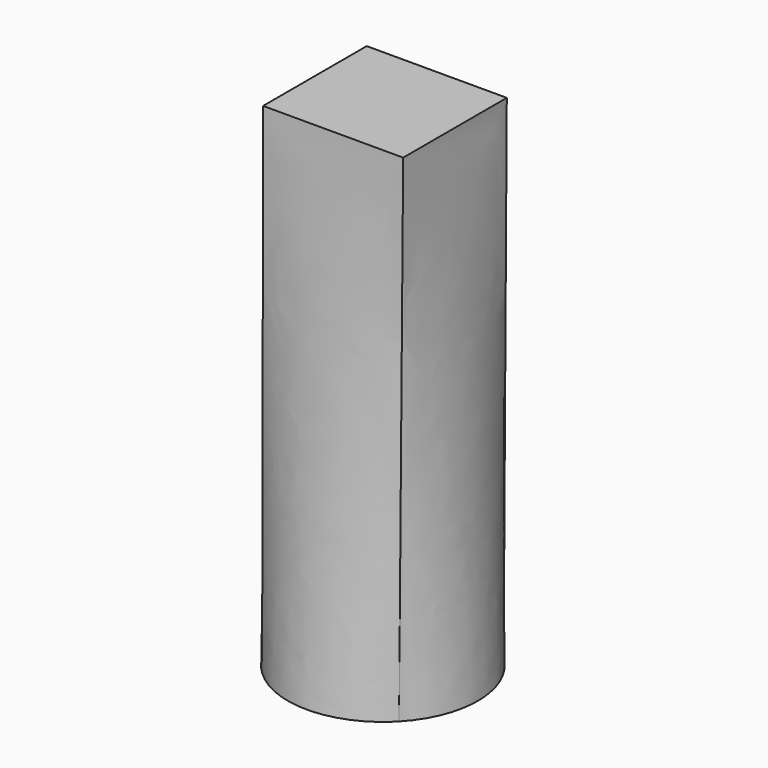
from build123d import *

# Parameters (mm, degrees)
F1_W = 28.2225450501
F1_H = 26.0982662439


# Not quite as in the source:
# - the arcs of a loft's sections are written as splines that run evenly, so that the points pair up as in the source's solid


with BuildPart() as f3:
    # F2 (on Top) → F3 section 0
    with BuildSketch(Plane.XY):
        with BuildLine():
            add(Edge.make_bspline(
                [(-13.8507158187, 13.2452200706), (-14.7176134451, 12.3386928401), (-15.4952067044, 11.3468081727), (-16.8419781891, 9.2303443707), (-17.4111231128, 8.1058175697), (-18.3191151563, 5.7672789435), (-18.6579398242, 4.5533249433), (-19.0922588016, 2.0825802209), (-19.1877423716, 0.8258505928), (-19.1316976481, -1.6821508917), (-18.9801707404, -2.9333607328), (-18.4359160833, -5.3822378889), (-18.0432017917, -6.5798446505), (-17.0316526023, -8.8754885024), (-16.412842717, -9.9734688283), (-14.9728722633, -12.0276590702), (-14.151747301, -12.9838181922), (-13.2452200706, -13.8507158187)],
                knots=[0, 0, 0, 0, 0.125, 0.125, 0.25, 0.25, 0.375, 0.375, 0.5, 0.5, 0.625, 0.625, 0.75, 0.75, 0.875, 0.875, 1, 1, 1, 1], degree=3))
            add(Edge.make_bspline(
                [(-13.2452200706, -13.8507158187), (-12.3386928401, -14.7176134451), (-11.3468081727, -15.4952067044), (-9.2303443707, -16.8419781891), (-8.1058175697, -17.4111231128), (-5.7672789435, -18.3191151563), (-4.5533249433, -18.6579398242), (-2.0825802209, -19.0922588016), (-0.8258505928, -19.1877423716), (1.6821508917, -19.1316976481), (2.9333607328, -18.9801707404), (5.3822378889, -18.4359160833), (6.5798446505, -18.0432017917), (8.8754885024, -17.0316526023), (9.9734688283, -16.412842717), (12.0276590702, -14.9728722633), (12.9838181922, -14.151747301), (13.8507158187, -13.2452200706)],
                knots=[0, 0, 0, 0, 0.125, 0.125, 0.25, 0.25, 0.375, 0.375, 0.5, 0.5, 0.625, 0.625, 0.75, 0.75, 0.875, 0.875, 1, 1, 1, 1], degree=3))
            add(Edge.make_bspline(
                [(13.8507158187, -13.2452200706), (14.7176134451, -12.3386928401), (15.4952067044, -11.3468081727), (16.8419781891, -9.2303443707), (17.4111231128, -8.1058175697), (18.3191151563, -5.7672789435), (18.6579398242, -4.5533249433), (19.0922588016, -2.0825802209), (19.1877423716, -0.8258505928), (19.1316976481, 1.6821508917), (18.9801707404, 2.9333607328), (18.4359160833, 5.3822378889), (18.0432017917, 6.5798446505), (17.0316526023, 8.8754885024), (16.412842717, 9.9734688283), (14.9728722633, 12.0276590702), (14.151747301, 12.9838181922), (13.2452200706, 13.8507158187)],
                knots=[0, 0, 0, 0, 0.125, 0.125, 0.25, 0.25, 0.375, 0.375, 0.5, 0.5, 0.625, 0.625, 0.75, 0.75, 0.875, 0.875, 1, 1, 1, 1], degree=3))
            add(Edge.make_bspline(
                [(13.2452200706, 13.8507158187), (12.3386928401, 14.7176134451), (11.3468081727, 15.4952067044), (9.2303443707, 16.8419781891), (8.1058175697, 17.4111231128), (5.7672789435, 18.3191151563), (4.5533249433, 18.6579398242), (2.0825802209, 19.0922588016), (0.8258505928, 19.1877423716), (-1.6821508917, 19.1316976481), (-2.9333607328, 18.9801707404), (-5.3822378889, 18.4359160833), (-6.5798446505, 18.0432017917), (-8.8754885024, 17.0316526023), (-9.9734688283, 16.412842717), (-12.0276590702, 14.9728722633), (-12.9838181922, 14.151747301), (-13.8507158187, 13.2452200706)],
                knots=[0, 0, 0, 0, 0.125, 0.125, 0.25, 0.25, 0.375, 0.375, 0.5, 0.5, 0.625, 0.625, 0.75, 0.75, 0.875, 0.875, 1, 1, 1, 1], degree=3))
        make_face()
    # F1 (on offset) → F3 section 1
    with BuildSketch(Plane.XY.offset(100)):
        with Locations((0.2276017331, 0.2276012674)):
            Rectangle(F1_W, F1_H)
    loft(ruled=True)


solid = f3.part
